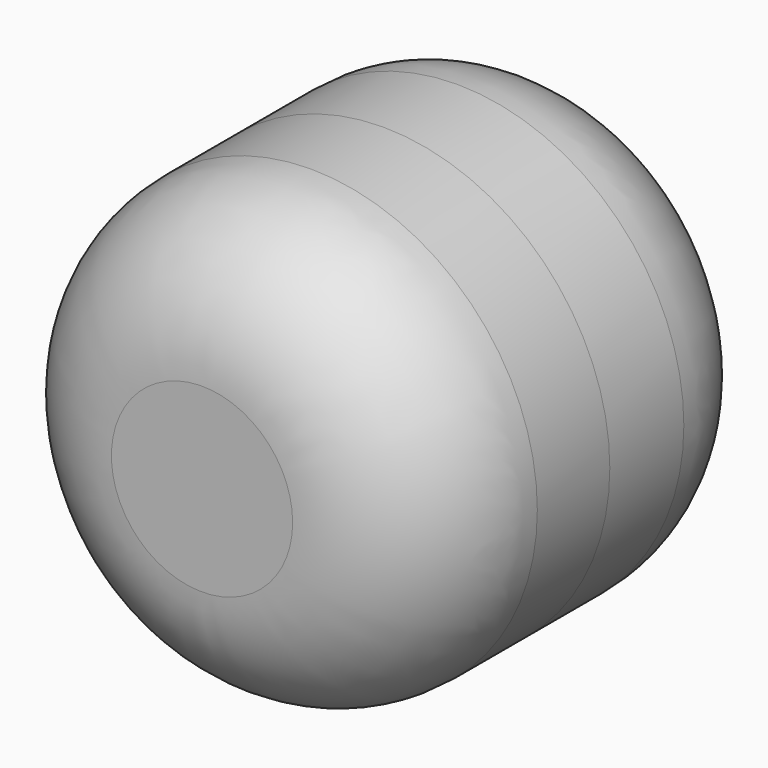
from build123d import *

# Parameters (mm, degrees)
F0_R     = 6.35
F1_DEPTH = 6.35
F2_R     = 6.35
F2_R_2   = 3.175
F3_DEPTH = 6.35


# Not quite as in the source:
# - a fillet or chamfer that OpenCascade refuses, or shapes differently, is made with other operations: its cross-section is extruded or revolved along the edge and cut away or added


with BuildPart() as f1:
    # F0 (on Front) → F1 (new body)
    with BuildSketch(Plane.XZ):
        Circle(F0_R)
    extrude(amount=F1_DEPTH)

    # F2 (on face) → F3 (join)
    with BuildSketch(Plane(origin=(0, 0, 0), x_dir=(-1, 0, 0), z_dir=(0, 1, 0))):
        Circle(F2_R)
        Circle(F2_R_2, mode=Mode.SUBTRACT)
    extrude(amount=F3_DEPTH)

    # F4: fillet of radius 3.81 on 2 edges, made by hand

    # F4_s1 → F4_t2 (revolve, cut)
    with BuildSketch(Plane.XY):
        with BuildLine():
            ThreePointArc((-6.35, 2.5932893377), (-5.4499355663, 5.0526337626), (-3.175, 6.35))
            Line((-3.175, 6.35), (-6.35, 6.35))
            Line((-6.35, 6.35), (-6.35, 2.5932893377))
        make_face()
    revolve(axis=Axis((0, 6.35, 0), (0, 1, 0)), mode=Mode.SUBTRACT)

    # F4_s3 → F4_t4 (revolve, cut)
    with BuildSketch(Plane.XY):
        with BuildLine():
            ThreePointArc((6.35, -2.54), (5.2340768363, -5.2340768363), (2.54, -6.35))
            Line((2.54, -6.35), (6.35, -6.35))
            Line((6.35, -6.35), (6.35, -2.54))
        make_face()
    revolve(axis=Axis((0, -6.35, 0), (0, -1, 0)), mode=Mode.SUBTRACT)


solid = f1.part
